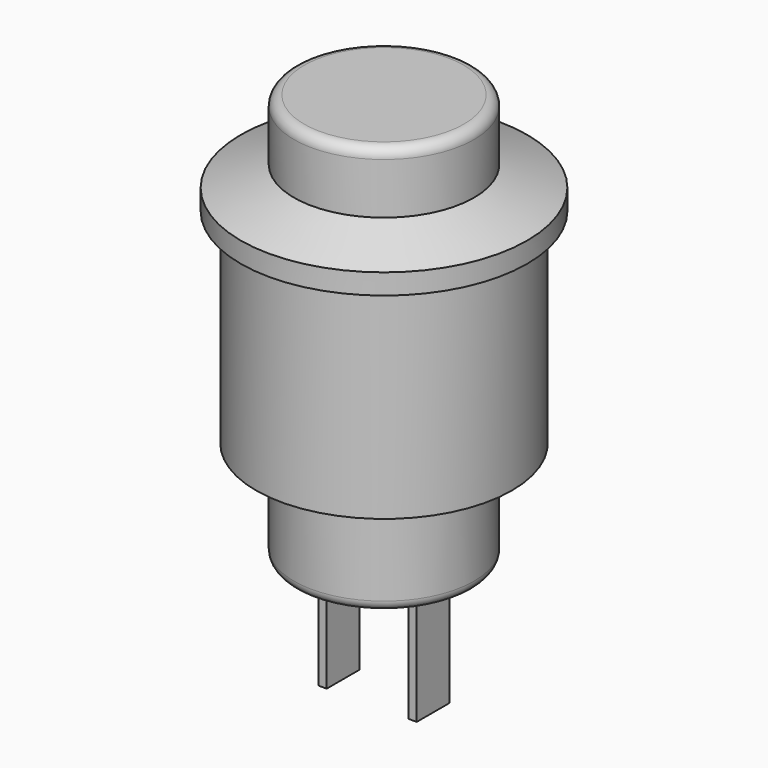
from build123d import *

# Parameters (mm, degrees)
F0_R      = 4.4
F1_DEPTH  = 20
F2_R      = 0.5
F4_R      = 7
F5_DEPTH  = 12
F6_W      = 0.4
F6_H      = 2
F7_DEPTH  = 5.8
F8_SIZE2  = 0.99999
F8_SIZE   = 2.59999
F9_R      = 7
F9_R_2    = 6.25
F10_DEPTH = 10


# Not quite as in the source:
# - a fillet or chamfer is up to 0.001 mm smaller than in the source, because OpenCascade refuses the exact size


with BuildPart() as f1:
    # F0 (on Top) → F1 (new body)
    with BuildSketch(Plane.XY):
        Circle(F0_R)
    extrude(amount=F1_DEPTH)

    # F2
    f2_edges = [f1.edges().sort_by_distance(p)[0] for p in [
        (-4.4, 0, 20),
        (-4.4, 0, 0),
    ]]
    fillet(f2_edges, radius=F2_R)

    # F4 (on offset) → F5 (join)
    with BuildSketch(Plane.XY.offset(17)):
        Circle(F4_R)
    extrude(amount=-F5_DEPTH)

    # F6 (on face) → F7 (join)
    with BuildSketch(Plane(origin=(0, 0, 0), x_dir=(1, 0, 0), z_dir=(0, 0, -1))):
        with Locations((-2.2, 0)):
            Rectangle(F6_W, F6_H)
        with Locations((2.2, 0)):
            Rectangle(F6_W, F6_H)
    extrude(amount=F7_DEPTH)

    # F8 (size 2.6 and 1 in the source; OpenCascade refuses exactly that, so slightly less here)
    f8_edges = [f1.edges().sort_by_distance(p)[0] for p in [
        (-7, 0, 17),
    ]]
    f8_side = f1.faces().sort_by_distance((-6.80201, 0, 17))[0]
    chamfer(f8_edges, length=F8_SIZE, length2=F8_SIZE2, reference=f8_side)

    # F9 (on face) → F10 (cut)
    with BuildSketch(Plane(origin=(0, 0, 5), x_dir=(1, 0, 0), z_dir=(0, 0, -1))):
        Circle(F9_R)
        Circle(F9_R_2, mode=Mode.SUBTRACT)
    extrude(amount=-F10_DEPTH, mode=Mode.SUBTRACT)


solid = f1.part
